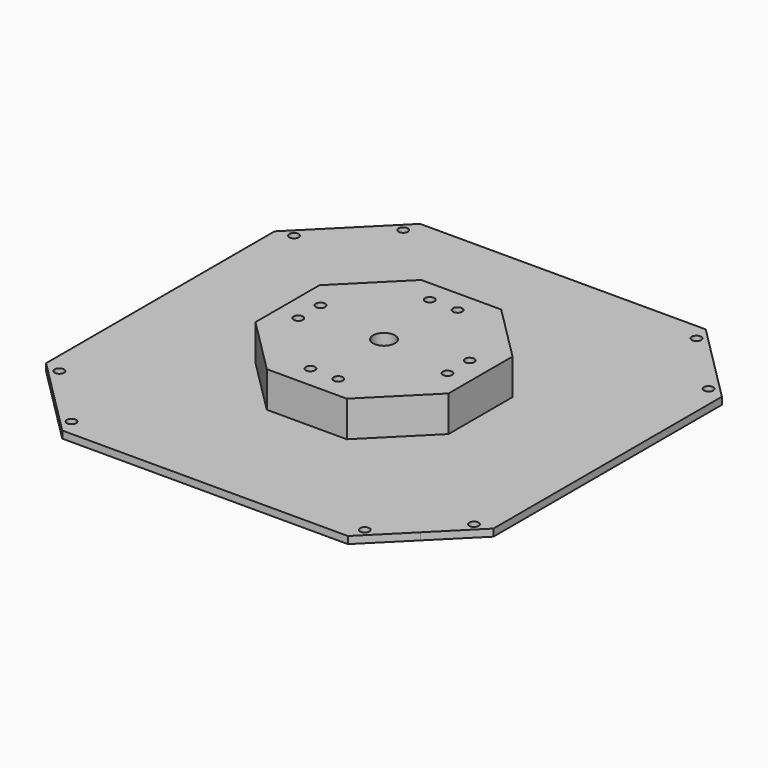
from build123d import *

# Parameters (mm, degrees)
F1_DEPTH = 4
F2_R     = 2.6
F3_DEPTH = 20
F4_R     = 2.6
F5_DEPTH = 4.001
F6_R     = 2.6
F6_R_2   = 6.1
F7_DEPTH = 20


# Not quite as in the source:
# - a feature names something its author has since deleted; it is built from what else it names


with BuildPart() as f1:
    # F0 (on Top) → F1 (new body)
    with BuildSketch(Plane.XY):
        Polygon((125.15, 79.85), (102.5, 102.5), (79.85, 125.15), (-79.9109665441, 125.15), (-102.530483272, 102.530483272), (-125.15, 79.9109665441), (-125.15, -79.85), (-102.5, -102.5), (-79.85, -125.15), (79.9109665441, -125.15), (102.530483272, -102.530483272), (125.15, -79.9109665441), align=None)
    extrude(amount=F1_DEPTH)

    # F2 (on face) → F3 (cut)
    with BuildSketch(Plane.XY.offset(4)):
        with Locations((-7.7781745931, 41.71930009)):
            Circle(F2_R)
        with Locations((-41.71930009, 7.7781745931)):
            Circle(F2_R)
        with Locations((7.7781745931, -41.71930009)):
            Circle(F2_R)
        with Locations((41.71930009, -7.7781745931)):
            Circle(F2_R)
        with Locations((41.71930009, 7.7781745931)):
            Circle(F2_R)
        with Locations((7.7781745931, 41.71930009)):
            Circle(F2_R)
        with Locations((-41.71930009, -7.7781745931)):
            Circle(F2_R)
        with Locations((-7.7781745931, -41.71930009)):
            Circle(F2_R)
    extrude(amount=-F3_DEPTH, mode=Mode.SUBTRACT)

    # F4 (on face) → F5 (cut, through all)
    with BuildSketch(Plane.XY.offset(4)):
        with Locations((-82.0243866176, 115.9655121146)):
            Circle(F4_R)
        with Locations((-115.9655121146, 82.0243866176)):
            Circle(F4_R)
        with Locations((82.0243866176, -115.9655121146)):
            Circle(F4_R)
        with Locations((115.9655121146, -82.0243866176)):
            Circle(F4_R)
        with Locations((82.0243866176, 115.9655121146)):
            Circle(F4_R)
        with Locations((115.9655121146, 82.0243866176)):
            Circle(F4_R)
        with Locations((-115.9655121146, -82.0243866176)):
            Circle(F4_R)
        with Locations((-82.0243866176, -115.9655121146)):
            Circle(F4_R)
    extrude(amount=-F5_DEPTH, mode=Mode.SUBTRACT)


with BuildPart() as f7:
    # F6 (on face) → F7 (new body)
    with BuildSketch(Plane.XY.offset(4)):
        Polygon((22.3675323681, 54), (-22.3675323681, 54), (-54, 22.3675323681), (-54, -22.3675323681), (-22.3675323681, -54), (22.3675323681, -54), (54, -22.3675323681), (54, 22.3675323681), align=None)
        with Locations((-7.7781745931, -41.71930009)):
            Circle(F6_R, mode=Mode.SUBTRACT)
        with Locations((-41.71930009, -7.7781745931)):
            Circle(F6_R, mode=Mode.SUBTRACT)
        with Locations((7.7781745931, -41.71930009)):
            Circle(F6_R, mode=Mode.SUBTRACT)
        with Locations((41.71930009, -7.7781745931)):
            Circle(F6_R, mode=Mode.SUBTRACT)
        with Locations((-41.71930009, 7.7781745931)):
            Circle(F6_R, mode=Mode.SUBTRACT)
        with Locations((-7.7781745931, 41.71930009)):
            Circle(F6_R, mode=Mode.SUBTRACT)
        Circle(F6_R_2, mode=Mode.SUBTRACT)
        with Locations((41.71930009, 7.7781745931)):
            Circle(F6_R, mode=Mode.SUBTRACT)
        with Locations((7.7781745931, 41.71930009)):
            Circle(F6_R, mode=Mode.SUBTRACT)
    extrude(amount=F7_DEPTH)


solid = Compound([f1.part, f7.part])
